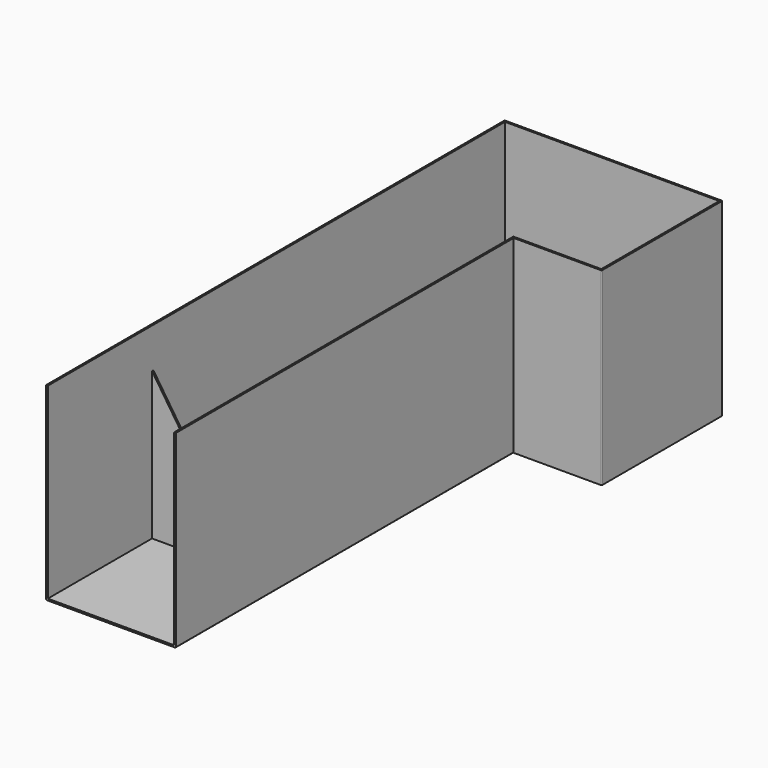
from build123d import *

# Parameters (mm, degrees)
F1_DEPTH  = 426
F3_DEPTH  = 4
F4_R      = 2
F7_DEPTH  = 4
F10_DEPTH = 4


# Not quite as in the source:
# - a feature names something its author has since deleted; it is built from what else it names


with BuildPart() as f1:
    # F0 (on Top) → F1 (new body)
    with BuildSketch(Plane.XY):
        Polygon((-200, -343), (0, -343), (0, 0), (-495, 0), (-495, -1303), (-491, -1303), (-491, -4), (-4, -4), (-4, -339), (-204, -339), (-204, -1303), (-200, -1303), align=None)
    extrude(amount=F1_DEPTH)

    # F2 (on Top) → F3 (join)
    with BuildSketch(Plane.XY):
        Polygon((0, 0), (-495, 0), (-495, -1303), (-200, -1303), (-200, -343), (0, -343), align=None)
    extrude(amount=-F3_DEPTH)

    # F4
    f4_edges = [f1.edges().sort_by_distance(p)[0] for p in [
        (-200, -823, -4),
        (-495, -651.5, -4),
        (-247.5, 0, -4),
        (0, -343, 211),
        (0, 0, 211),
    ]]
    fillet(f4_edges, radius=F4_R)

    # F6 (on offset) → F7 (join)
    with BuildSketch(Plane.XZ.offset(1003)):
        Polygon((-491, 0), (-269, 0), (-491, 335), align=None)
    extrude(amount=F7_DEPTH)

    # F9 (on offset) → F10 (join)
    with BuildSketch(Plane.XZ.offset(403)):
        Polygon((-204, 335), (-426, 0), (-204, 0), align=None)
    extrude(amount=F10_DEPTH)


solid = f1.part
